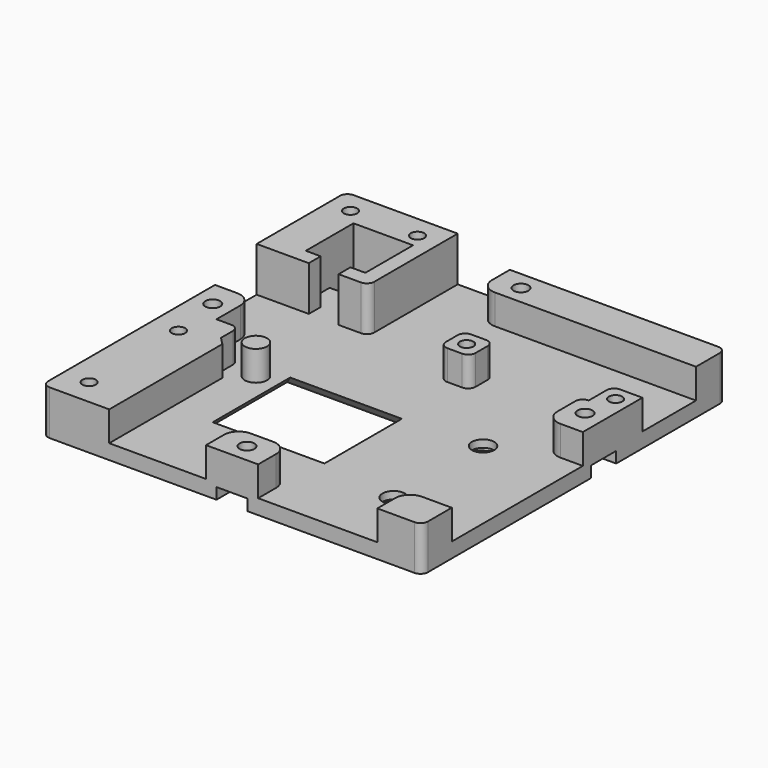
from build123d import *

# Parameters (mm, degrees)
F1_DEPTH         = 2
F2_W             = 5
F2_H             = 5
F3_DEPTH         = 4
F4_DEPTH         = 6
F5_R             = 1
F7_D             = 2
F7_CBORE_D       = 4.2
F7_CBORE_DEPTH   = 1.5
F2_W_2           = 15
F2_H_2           = 13
F8_DEPTH         = 25
F9_SIZE          = 1.99999
F10_R            = 1.5
F11_DEPTH        = 4
F14_DEPTH        = 6
F16_DEPTH        = 1.5
F18_DEPTH        = 1
F19_D            = 3
F20_W            = 4
F20_H            = 4
F21_DEPTH        = 4
F22_R            = 0.99999
F24_D            = 1.8
F24_DEPTH        = 5
F24_TIP          = 0.5407745571
F24_ON_F13_D     = 1.8
F24_ON_F13_DEPTH = 5
F24_ON_F13_TIP   = 0.5407745571
F24_ON_F23_D     = 1.8
F24_ON_F23_DEPTH = 5
F24_ON_F23_TIP   = 0.5407745571
F25_DEPTH        = 3
F27_DEPTH        = 2.5
F28_SIZE         = 1.99999
F29_R            = 0.99999
F30_DEPTH        = 1
F31_DEPTH        = 1
F32_DEPTH        = 1
F33_DEPTH        = 1
F34_R            = 2
F36_D            = 1.8
F36_DEPTH        = 5
F36_TIP          = 0.5407745571


# Not quite as in the source:
# - a fillet or chamfer is up to 0.001 mm smaller than in the source, because OpenCascade refuses the exact size
# - a feature names something its author has since deleted; it is built from what else it names


with BuildPart() as f1:
    # F0 (on Top) → F1 (new body)
    with BuildSketch(Plane.XY):
        with BuildLine():
            Line((-24.5, -25.5), (24.5, -25.5))
            ThreePointArc((24.5, -25.5), (25.2071067812, -25.2071067812), (25.5, -24.5))
            Line((25.5, -24.5), (25.5, 24.5))
            ThreePointArc((25.5, 24.5), (25.2071067812, 25.2071067812), (24.5, 25.5))
            Line((24.5, 25.5), (-24.5, 25.5))
            ThreePointArc((-24.5, 25.5), (-25.2071067812, 25.2071067812), (-25.5, 24.5))
            Line((-25.5, 24.5), (-25.5, -24.5))
            ThreePointArc((-25.5, -24.5), (-25.2071067812, -25.2071067812), (-24.5, -25.5))
        make_face()
    extrude(amount=F1_DEPTH)

    # F2 (on face) → F3 (join)
    with BuildSketch(Plane.XY.offset(2)):
        with Locations((-23, 0)):
            Rectangle(F2_W, F2_H)
        with Locations((0, 23)):
            Rectangle(F2_W, F2_H)
        with Locations((23, 5)):
            Rectangle(F2_W, F2_H)
        with Locations((0, -23)):
            Rectangle(F2_W, F2_H)
    extrude(amount=F3_DEPTH)

    # F2 (on face) → F4 (join)
    with BuildSketch(Plane.XY.offset(2)):
        with BuildLine():
            Line((-25.5, 24.5), (-25.5, 10.5))
            Line((-25.5, 10.5), (-10.5, 10.5))
            Line((-10.5, 10.5), (-10.5, 25.5))
            Line((-10.5, 25.5), (-24.5, 25.5))
            ThreePointArc((-24.5, 25.5), (-25.2071067812, 25.2071067812), (-25.5, 24.5))
        make_face()
    extrude(amount=F4_DEPTH)

    # F5
    f5_edges = [f1.edges().sort_by_distance(p)[0] for p in [
        (-10.5, 10.5, 5),
    ]]
    fillet(f5_edges, radius=F5_R)

    # F7 (through all)
    with Locations(Plane(origin=(0, 0, 0), x_dir=(1, 0, 0), z_dir=(0, 0, -1))):
        with Locations((-23, 0), (0, 23), (23, -5), (0, -23)):
            CounterBoreHole(F7_D / 2, F7_CBORE_D / 2, F7_CBORE_DEPTH)

    # F2 (on face) → F8 (cut)
    with BuildSketch(Plane.XY.offset(2)):
        with Locations((-3.5, -8.5)):
            Rectangle(F2_W_2, F2_H_2)
    extrude(amount=-F8_DEPTH, mode=Mode.SUBTRACT)

    # F9 (size 2 in the source; OpenCascade refuses exactly that, so slightly less here)
    f9_edges = [f1.edges().sort_by_distance(p)[0] for p in [
        (-11, -8.5, 0),
        (-3.5, -15, 0),
        (4, -8.5, 0),
        (-3.5, -2, 0),
    ]]
    chamfer(f9_edges, length=F9_SIZE)

    # F10 (on face) → F11 (join)
    with BuildSketch(Plane.XY.offset(2)):
        with BuildLine():
            Line((-24.5, -25.5), (-16.5, -25.5))
            Line((-16.5, -25.5), (-16.5, -6.5))
            Line((-16.5, -6.5), (-17.5, -5.5))
            Line((-17.5, -5.5), (-17.5, -3.5))
            ThreePointArc((-17.5, -3.5), (-17.7928932188, -2.7928932188), (-18.5, -2.5))
            Line((-18.5, -2.5), (-20.5, -2.5))
            Line((-20.5, -2.5), (-25.5, -2.5))
            Line((-25.5, -2.5), (-25.5, -24.5))
            ThreePointArc((-25.5, -24.5), (-25.2071067812, -25.2071067812), (-24.5, -25.5))
        make_face()
        with Locations((-14, -4)):
            Circle(F10_R)
    extrude(amount=F11_DEPTH)

    # F13 (on face) → F14 (cut)
    with BuildSketch(Plane.XY.offset(8)):
        Polygon((-14.5, 12.5), (-12.5, 12.5), (-12.5, 20.5), (-23.5, 20.5), (-23.5, 12.5), (-18.5, 12.5), (-18.5, 10.5), (-14.5, 10.5), align=None)
    extrude(amount=-F14_DEPTH, mode=Mode.SUBTRACT)

    # F15 (on face) → F16 (cut)
    with BuildSketch(Plane(origin=(0, 0, 0), x_dir=(1, 0, 0), z_dir=(0, 0, -1))):
        with BuildLine():
            ThreePointArc((-2.1, 23), (0, 25.1), (2.1, 23))
            Line((2.1, 23), (2.1, 25.5))
            Line((2.1, 25.5), (-2.1, 25.5))
            Line((-2.1, 25.5), (-2.1, 23))
        make_face()
        with BuildLine():
            Line((25.5, -7.1), (25.5, -2.9))
            Line((25.5, -2.9), (23, -2.9))
            ThreePointArc((23, -2.9), (24.4849242405, -3.5150757595), (25.1, -5))
            ThreePointArc((25.1, -5), (24.4849242405, -6.4849242405), (23, -7.1))
            Line((23, -7.1), (25.5, -7.1))
        make_face()
        with BuildLine():
            Line((-23, 2.1), (-25.5, 2.1))
            Line((-25.5, 2.1), (-25.5, -2.1))
            Line((-25.5, -2.1), (-23, -2.1))
            ThreePointArc((-23, -2.1), (-25.1, 0), (-23, 2.1))
        make_face()
        with BuildLine():
            Line((-2.1, -25.5), (2.1, -25.5))
            Line((2.1, -25.5), (2.1, -23))
            ThreePointArc((2.1, -23), (0, -25.1), (-2.1, -23))
            Line((-2.1, -23), (-2.1, -25.5))
        make_face()
    extrude(amount=-F16_DEPTH, mode=Mode.SUBTRACT)

    # F17 (on face) → F18 (cut)
    with BuildSketch(Plane(origin=(0, 0, 0), x_dir=(1, 0, 0), z_dir=(0, 0, -1))):
        Polygon((17.25, 18.0877132403), (14.5, 19.6754264805), (11.75, 18.0877132403), (11.75, 14.9122867597), (14.5, 13.3245735195), (17.25, 14.9122867597), align=None)
        Polygon((17.25, -0.0877132403), (17.25, 3.0877132403), (14.5, 4.6754264805), (11.75, 3.0877132403), (11.75, -0.0877132403), (14.5, -1.6754264805), align=None)
    extrude(amount=-F18_DEPTH, mode=Mode.SUBTRACT)

    # F19 (through all)
    with Locations(Plane(origin=(0, 0, 0), x_dir=(1, 0, 0), z_dir=(0, 0, -1))):
        with Locations((14.5, 16.5), (14.5, 1.5)):
            Hole(F19_D / 2)

    # F20 (on face) → F21 (join)
    with BuildSketch(Plane.XY.offset(2)):
        with Locations((23.5, 9.5)):
            Rectangle(F20_W, F20_H)
        with Locations((3.5, 9.5)):
            Rectangle(F20_W, F20_H)
        with BuildLine():
            Line((2.5, 20.5), (25.5, 20.5))
            Line((25.5, 20.5), (25.5, 24.5))
            ThreePointArc((25.5, 24.5), (25.2071067812, 25.2071067812), (24.5, 25.5))
            Line((24.5, 25.5), (2.5, 25.5))
            Line((2.5, 25.5), (2.5, 20.5))
        make_face()
        with BuildLine():
            Line((25.5, -24.5), (25.5, -20.5))
            Line((25.5, -20.5), (20.5, -20.5))
            Line((20.5, -20.5), (20.5, -25.5))
            Line((20.5, -25.5), (24.5, -25.5))
            ThreePointArc((24.5, -25.5), (25.2071067812, -25.2071067812), (25.5, -24.5))
        make_face()
    extrude(amount=F21_DEPTH)

    # F22 (radius 1 in the source; OpenCascade refuses exactly that, so slightly less here)
    f22_edges = [f1.edges().sort_by_distance(p)[0] for p in [
        (5.5, 7.5, 4),
        (1.5, 7.5, 4),
        (1.5, 11.5, 4),
        (20.5, 7.5, 4),
        (5.5, 11.5, 4),
        (21.5, 11.5, 4),
    ]]
    fillet(f22_edges, radius=F22_R)

    # F24
    with Locations(Plane.XY.offset(6)):
        with Locations((-22, -22), (-22, -7)):
            Hole(F24_D / 2, depth=F24_DEPTH)
            with Locations((0, 0, -(F24_DEPTH + F24_TIP / 2))):  # 118° drill point
                Cone(0, F24_D / 2, F24_TIP, mode=Mode.SUBTRACT)

    # F24 on F13
    with Locations(Plane.XY.offset(8)):
        with Locations((-22.5, 22.5), (-13.5, 22.5)):
            Hole(F24_ON_F13_D / 2, depth=F24_ON_F13_DEPTH)
            with Locations((0, 0, -(F24_ON_F13_DEPTH + F24_ON_F13_TIP / 2))):  # 118° drill point
                Cone(0, F24_ON_F13_D / 2, F24_ON_F13_TIP, mode=Mode.SUBTRACT)

    # F24 on F23
    with Locations(Plane.XY.offset(6)):
        with Locations((3.5, 9.5), (23.5, 9.5)):
            Hole(F24_ON_F23_D / 2, depth=F24_ON_F23_DEPTH)
            with Locations((0, 0, -(F24_ON_F23_DEPTH + F24_ON_F23_TIP / 2))):  # 118° drill point
                Cone(0, F24_ON_F23_D / 2, F24_ON_F23_TIP, mode=Mode.SUBTRACT)

    # F25 (add): a face of the model
    f25_faces = [f1.faces().sort_by_distance(p)[0] for p in [
        (-23.5, 16.5, 5),
    ]]
    extrude(f25_faces, amount=F25_DEPTH)

    # F26 (on face) → F27 (cut)
    with BuildSketch(Plane(origin=(0, 0, 0), x_dir=(1, 0, 0), z_dir=(0, 0, -1))):
        with BuildLine():
            Line((-20.5, -21.5), (-21.5, -21.5))
            Line((-21.5, -21.5), (-25.5, -21.5))
            Line((-25.5, -21.5), (-25.5, -24.5))
            ThreePointArc((-25.5, -24.5), (-25.2071067812, -25.2071067812), (-24.5, -25.5))
            Line((-24.5, -25.5), (-21.5, -25.5))
            Line((-21.5, -25.5), (-21.5, -24.5))
            Line((-21.5, -24.5), (-15, -24.5))
            Line((-15, -24.5), (-15, -21))
            Line((-15, -21), (-15, -18.5))
            Line((-15, -18.5), (-20.5, -18.5))
            Line((-20.5, -18.5), (-20.5, -21.5))
        make_face()
    extrude(amount=-F27_DEPTH, mode=Mode.SUBTRACT)

    # F28 (size 2 in the source; OpenCascade refuses exactly that, so slightly less here)
    f28_edges = [f1.edges().sort_by_distance(p)[0] for p in [
        (-17.75, 18.5, 2),
    ]]
    chamfer(f28_edges, length=F28_SIZE)

    # F29 (radius 1 in the source; OpenCascade refuses exactly that, so slightly less here)
    f29_edges = [f1.edges().sort_by_distance(p)[0] for p in [
        (-25.5, 21.5, 1.25),
        (-21.5, 24.5, 1.25),
        (-15, 24.5, 1.25),
    ]]
    fillet(f29_edges, radius=F29_R)

    # F30 (add): faces of the model
    f30_faces = [f1.faces().sort_by_distance(p)[0] for p in [
        (-2.5, 23, 4),
        (-2.5, -23, 4),
        (20.5, -23, 4),
    ]]
    extrude(f30_faces, amount=F30_DEPTH)

    # F31 (add): a face of the model
    f31_faces = [f1.faces().sort_by_distance(p)[0] for p in [
        (2.5, -23, 4),
    ]]
    extrude(f31_faces, amount=F31_DEPTH)

    # F32 (add): a face of the model
    f32_faces = [f1.faces().sort_by_distance(p)[0] for p in [
        (23, 2.5, 4),
    ]]
    extrude(f32_faces, amount=F32_DEPTH)

    # F33 (add): a face of the model
    f33_faces = [f1.faces().sort_by_distance(p)[0] for p in [
        (-23, 2.5, 4),
    ]]
    extrude(f33_faces, amount=F33_DEPTH)

    # F34
    f34_edges = [f1.edges().sort_by_distance(p)[0] for p in [
        (19.5, -20.5, 4),
        (20.5, 1.5, 4),
        (3.5, -20.5, 4),
        (-3.5, -20.5, 4),
        (-3.5, 20.5, 4),
        (-20.5, 3.5, 4),
    ]]
    fillet(f34_edges, radius=F34_R)

    # F36
    with Locations(Plane(origin=(0, 0, 0), x_dir=(1, 0, 0), z_dir=(0, 0, -1))):
        with Locations((-23, -18.5), (-23, 18.5), (23, -23), (23, 23)):
            Hole(F36_D / 2, depth=F36_DEPTH)
            with Locations((0, 0, -(F36_DEPTH + F36_TIP / 2))):  # 118° drill point
                Cone(0, F36_D / 2, F36_TIP, mode=Mode.SUBTRACT)


solid = f1.part
